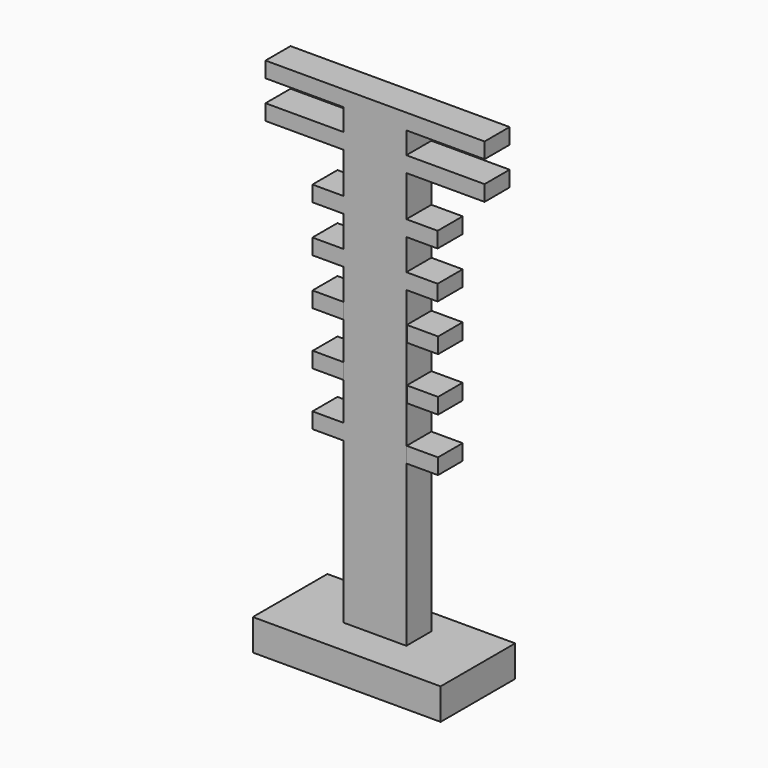
from build123d import *

# Parameters (mm, degrees)
F0_W      = 152.4
F0_H      = 75.6477481976
F1_DEPTH  = 25.4
F2_W      = 50.8
F2_H      = 25.4
F3_DEPTH  = 381
F4_W      = 25.4
F4_H      = 12.7
F5_DEPTH  = 63.5
F6_W      = 25.4
F6_H      = 12.7
F7_DEPTH  = 63.5
F8_W      = 25.4
F8_H      = 12.7
F9_DEPTH  = 63.5
F10_W     = 25.4
F10_H     = 12.7
F11_DEPTH = 63.5
F12_W     = 25.4
F12_H     = 12.7
F13_DEPTH = 25.4
F14_W     = 25.4
F14_H     = 12.7
F18_DEPTH = 25.4
F15_W     = 24.92688122
F15_H     = 12.7
F19_DEPTH = 25.4
F16_W     = 24.9687274059
F16_H     = 12.7
F20_DEPTH = 25.4
F17_W     = 25.0190113743
F17_H     = 12.7
F21_DEPTH = 25.4
F22_W     = 25.4
F22_H     = 12.7
F27_DEPTH = 25.4
F23_W     = 25.320323884
F23_H     = 12.7
F28_DEPTH = 25.4
F24_W     = 25.3337946793
F24_H     = 12.7
F29_DEPTH = 25.4
F25_W     = 25.1309572571
F25_H     = 12.7
F30_DEPTH = 25.4
F26_W     = 25.4
F26_H     = 12.7
F31_DEPTH = 25.4


with BuildPart() as f1:
    # F0 (on Top) → F1 (new body)
    with BuildSketch(Plane.XY):
        with Locations((-1.49496e-05, -37.8238740988)):
            Rectangle(F0_W, F0_H)
    extrude(amount=F1_DEPTH)

    # F2 (on face) → F3 (join)
    with BuildSketch(Plane.XY.offset(25.4)):
        with Locations((-0.9335875511, -33.0558609421)):
            Rectangle(F2_W, F2_H)
    extrude(amount=F3_DEPTH)

    # F4 (on face) → F5 (join)
    with BuildSketch(Plane.YZ.offset(24.4664124489)):
        with Locations((-33.0558609421, 400.05)):
            Rectangle(F4_W, F4_H)
    extrude(amount=F5_DEPTH)

    # F6 (on face) → F7 (join)
    with BuildSketch(Plane.YZ.offset(24.4664124489)):
        with Locations((-33.0558609421, 369.57)):
            Rectangle(F6_W, F6_H)
    extrude(amount=F7_DEPTH)

    # F8 (on face) → F9 (join)
    with BuildSketch(Plane(origin=(-26.3335875511, 0, 0), x_dir=(0, -1, 0), z_dir=(-1, 0, 0))):
        with Locations((33.0558609421, 400.05)):
            Rectangle(F8_W, F8_H)
    extrude(amount=F9_DEPTH)

    # F10 (on face) → F11 (join)
    with BuildSketch(Plane(origin=(-26.3335875511, 0, 0), x_dir=(0, -1, 0), z_dir=(-1, 0, 0))):
        with Locations((33.0558609421, 369.57)):
            Rectangle(F10_W, F10_H)
    extrude(amount=F11_DEPTH)

    # F12 (on face) → F13 (join)
    with BuildSketch(Plane.YZ.offset(24.4664124489)):
        with Locations((-33.0558609421, 323.85)):
            Rectangle(F12_W, F12_H)
    extrude(amount=F13_DEPTH)

    # F14 (on face) → F18 (join)
    with BuildSketch(Plane.YZ.offset(24.4664124489)):
        with Locations((-33.0558609421, 286.004)):
            Rectangle(F14_W, F14_H)
    extrude(amount=F18_DEPTH)

    # F15 (on face) → F19 (join)
    with BuildSketch(Plane.YZ.offset(24.4664124489)):
        with Locations((-32.8193015521, 248.158)):
            Rectangle(F15_W, F15_H)
    extrude(amount=F19_DEPTH)

    # F16 (on face) → F20 (join)
    with BuildSketch(Plane.YZ.offset(24.4664124489)):
        with Locations((-32.840224645, 204.978)):
            Rectangle(F16_W, F16_H)
    extrude(amount=F20_DEPTH)

    # F17 (on face) → F21 (join)
    with BuildSketch(Plane.YZ.offset(24.4664124489)):
        with Locations((-32.8653666293, 161.798)):
            Rectangle(F17_W, F17_H)
    extrude(amount=F21_DEPTH)

    # F22 (on face) → F27 (join)
    with BuildSketch(Plane(origin=(-26.3335875511, 0, 0), x_dir=(0, -1, 0), z_dir=(-1, 0, 0))):
        with Locations((33.0558609421, 323.85)):
            Rectangle(F22_W, F22_H)
    extrude(amount=F27_DEPTH)

    # F23 (on face) → F28 (join)
    with BuildSketch(Plane(origin=(-26.3335875511, 0, 0), x_dir=(0, -1, 0), z_dir=(-1, 0, 0))):
        with Locations((33.0956990001, 286.004)):
            Rectangle(F23_W, F23_H)
    extrude(amount=F28_DEPTH)

    # F24 (on face) → F29 (join)
    with BuildSketch(Plane(origin=(-26.3335875511, 0, 0), x_dir=(0, -1, 0), z_dir=(-1, 0, 0))):
        with Locations((33.0227582817, 248.158)):
            Rectangle(F24_W, F24_H)
    extrude(amount=F29_DEPTH)

    # F25 (on face) → F30 (join)
    with BuildSketch(Plane(origin=(-26.3335875511, 0, 0), x_dir=(0, -1, 0), z_dir=(-1, 0, 0))):
        with Locations((32.9213395706, 204.978)):
            Rectangle(F25_W, F25_H)
    extrude(amount=F30_DEPTH)

    # F26 (on face) → F31 (join)
    with BuildSketch(Plane(origin=(-26.3335875511, 0, 0), x_dir=(0, -1, 0), z_dir=(-1, 0, 0))):
        with Locations((33.0558609421, 161.798)):
            Rectangle(F26_W, F26_H)
    extrude(amount=F31_DEPTH)


solid = f1.part
